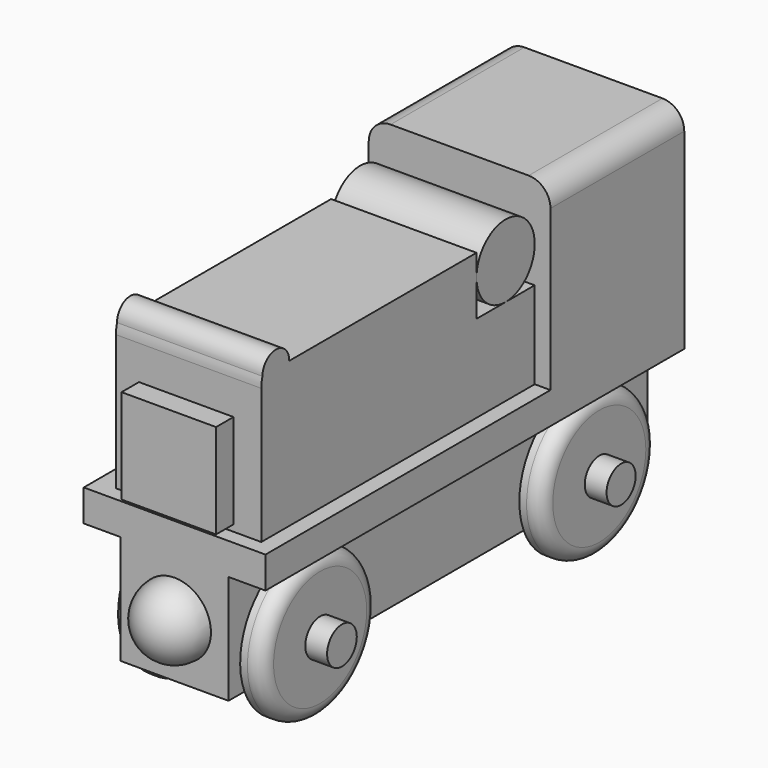
from build123d import *

# Parameters (mm, degrees)
F0_W         = 20
F0_H         = 20
F1_DEPTH     = 5
F2_W         = 20
F2_H         = 8
F3_DEPTH     = 27
F4_W         = 20
F4_H         = 12
F5_DEPTH     = 37
F6_W         = 24.9961130321
F6_H         = 4.3615074828
F7_DEPTH     = 65
F8_W         = 24.9961130321
F8_H         = 4.3615074828
F9_DEPTH     = 7
F10_W        = 24.9961130321
F10_H        = 23
F11_DEPTH    = 25
F12_R        = 5.00513233
F13_DEPTH    = 20
F14_W        = 14.829759486
F14_H        = 72
F15_DEPTH    = 15
F17_DEPTH    = 20
F18_T1_DEPTH = 26.8793659776
F19_R        = 10
F20_DEPTH    = 3
F22_DEPTH    = 3
F25_R        = 2.5526009998
F26_DEPTH    = 3
F27_R        = 2.5
F28_DEPTH    = 3
F29_R        = 2.5
F30_DEPTH    = 3
F31_R        = 2.5
F32_DEPTH    = 3
F33_R        = 2
F34_R        = 3
F35_W        = 13
F35_H        = 13
F36_DEPTH    = 3


# Not quite as in the source:
# - a fillet or chamfer that OpenCascade refuses, or shapes differently, is made with other operations: its cross-section is extruded or revolved along the edge and cut away or added


with BuildPart() as f1:
    # F0 (on Front) → F1 (new body, symmetric)
    with BuildSketch(Plane.XZ):
        with Locations((0.3240229562, 2.5902625751)):
            Rectangle(F0_W, F0_H)
    extrude(amount=F1_DEPTH, both=True)

    # F2 (on face) → F3 (join)
    with BuildSketch(Plane(origin=(0, 5, 0), x_dir=(-1, 0, 0), z_dir=(0, 1, 0))):
        with Locations((-0.3240229562, 8.5902625751)):
            Rectangle(F2_W, F2_H)
    extrude(amount=F3_DEPTH)

    # F4 (on face) → F5 (join)
    with BuildSketch(Plane(origin=(0, 5, 0), x_dir=(-1, 0, 0), z_dir=(0, 1, 0))):
        with Locations((-0.3240229562, -1.4097374249)):
            Rectangle(F4_W, F4_H)
    extrude(amount=F5_DEPTH)

    # F6 (on Front) → F7 (join)
    with BuildSketch(Plane.XZ):
        with Locations((0, -9.5765283331)):
            Rectangle(F6_W, F6_H)
    extrude(amount=-F7_DEPTH)

    # F8 (on face) → F9 (join)
    with BuildSketch(Plane.XZ):
        with Locations((0, -9.5765283331)):
            Rectangle(F8_W, F8_H)
    extrude(amount=F9_DEPTH)

    # F10 (on face) → F11 (join)
    with BuildSketch(Plane.XY.offset(-7.3957745917)):
        with Locations((0, 53.5)):
            Rectangle(F10_W, F10_H)
    extrude(amount=F11_DEPTH)

    # F14 (on face) → F15 (join)
    with BuildSketch(Plane(origin=(0, 0, -11.7572820745), x_dir=(1, 0, 0), z_dir=(0, 0, -1))):
        with Locations((0, -29)):
            Rectangle(F14_W, F14_H)
    extrude(amount=F15_DEPTH)

    # F16 (on face) → F17 (join)
    with BuildSketch(Plane.YZ.offset(10.3240229562)):
        with BuildLine():
            ThreePointArc((-0.1930287134, 12.5902625751), (-2.5, 14.8972338617), (-4.8069712866, 12.5902625751))
            Line((-4.8069712866, 12.5902625751), (-0.1930287134, 12.5902625751))
        make_face()
    extrude(amount=-F17_DEPTH)

    # F18: fillet of radius 5 on 1 edges, made by hand

    # F18_s2 → F18_t1 (cut)
    with BuildSketch(Plane.YZ.offset(-13.1156600326)):
        with BuildLine():
            ThreePointArc((-4.8069712866, 12.5902625751), (-4.951507671, 11.9090632481), (-5, 11.2143893796))
            Line((-5, 11.2143893796), (-5, 12.5902625751))
            Line((-5, 12.5902625751), (-4.8069712866, 12.5902625751))
        make_face()
    extrude(amount=F18_T1_DEPTH, mode=Mode.SUBTRACT)

    # F19 (on face) → F20 (join)
    with BuildSketch(Plane.YZ.offset(7.414879743)):
        with Locations((5, -22.9782015085)):
            Circle(F19_R)
        with Locations((53, -22.9782015085)):
            Circle(F19_R)
    extrude(amount=F20_DEPTH)

    # F21 (on face) → F22 (join)
    with BuildSketch(Plane(origin=(-7.414879743, 0, 0), x_dir=(0, -1, 0), z_dir=(-1, 0, 0))):
        with BuildLine():
            ThreePointArc((-43, -22.9782015085), (-54.9255761518, -13.1653448152), (-62.2584312967, -26.7572820745))
            ThreePointArc((-62.2584312967, -26.7572820745), (-53, -32.9782015085), (-43.7415687033, -26.7572820745))
            ThreePointArc((-43.7415687033, -26.7572820745), (-43.1871433067, -24.9037776604), (-43, -22.9782015085))
        make_face()
        with BuildLine():
            ThreePointArc((5, -22.9782015085), (-6.9255761518, -13.1653448152), (-14.2584312967, -26.7572820745))
            ThreePointArc((-14.2584312967, -26.7572820745), (-5, -32.9782015085), (4.2584312967, -26.7572820745))
            ThreePointArc((4.2584312967, -26.7572820745), (4.8128566933, -24.9037776604), (5, -22.9782015085))
        make_face()
    extrude(amount=F22_DEPTH)

    # F23 (on face) → F24 (revolve)
    with BuildSketch(Plane.XZ.offset(7)):
        with BuildLine():
            Line((0, -24.2572820745), (0, -14.2572820745))
            ThreePointArc((0, -14.2572820745), (-5, -19.2572820745), (0, -24.2572820745))
        make_face()
    revolve(axis=Axis((0, -7, -19.2572820745), (0, 0, -1)))

    # F25 (on face) → F26 (join)
    with BuildSketch(Plane.YZ.offset(10.414879743)):
        with Locations((5, -22.9782015085)):
            Circle(F25_R)
    extrude(amount=F26_DEPTH)

    # F27 (on face) → F28 (join)
    with BuildSketch(Plane.YZ.offset(10.414879743)):
        with Locations((53, -22.9782015085)):
            Circle(F27_R)
    extrude(amount=F28_DEPTH)

    # F29 (on face) → F30 (join)
    with BuildSketch(Plane(origin=(-10.414879743, 0, 0), x_dir=(0, -1, 0), z_dir=(-1, 0, 0))):
        with Locations((-5, -22.9782015085)):
            Circle(F29_R)
    extrude(amount=F30_DEPTH)

    # F31 (on face) → F32 (join)
    with BuildSketch(Plane(origin=(-10.414879743, 0, 0), x_dir=(0, -1, 0), z_dir=(-1, 0, 0))):
        with Locations((-53, -22.9782015085)):
            Circle(F31_R)
    extrude(amount=F32_DEPTH)

    # F33
    f33_edges = [f1.edges().sort_by_distance(p)[0] for p in [
        (-10.41488, 63, -22.978202),
        (-10.41488, 15, -22.978202),
        (10.41488, 43, -22.978202),
        (10.41488, -5, -22.978202),
    ]]
    fillet(f33_edges, radius=F33_R)

    # F34
    f34_edges = [f1.edges().sort_by_distance(p)[0] for p in [
        (12.498057, 53.5, 17.604225),
        (-12.498057, 53.5, 17.604225),
    ]]
    fillet(f34_edges, radius=F34_R)

    # F35 (on face) → F36 (join)
    with BuildSketch(Plane.XZ.offset(5)):
        Rectangle(F35_W, F35_H)
    extrude(amount=F36_DEPTH)


with BuildPart() as f13:
    # F12 (on face) → F13 (new body)
    with BuildSketch(Plane.YZ.offset(10.3240229562)):
        with Locations((37, 9.5953949051)):
            Circle(F12_R)
    extrude(amount=-F13_DEPTH)


solid = Compound([f1.part, f13.part])
